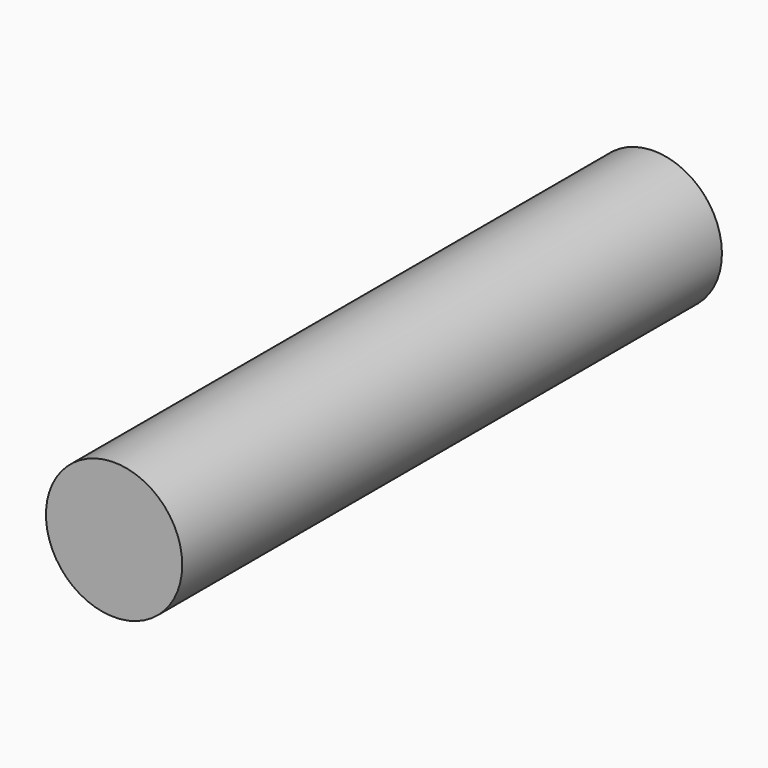
from build123d import *

# Parameters (mm, degrees)
F0_R     = 1.01
F1_DEPTH = 10


# Not quite as in the source:
# - the program builds the solid bodies; features that only make, move or delete a surface that nothing else refers to are left out


with BuildPart() as f1:
    # F0 (on Front) → F1 (new body)
    with BuildSketch(Plane.XZ):
        with Locations((-10.3005478159, 24.202408269)):
            Circle(F0_R)
    extrude(amount=-F1_DEPTH)


solid = f1.part
